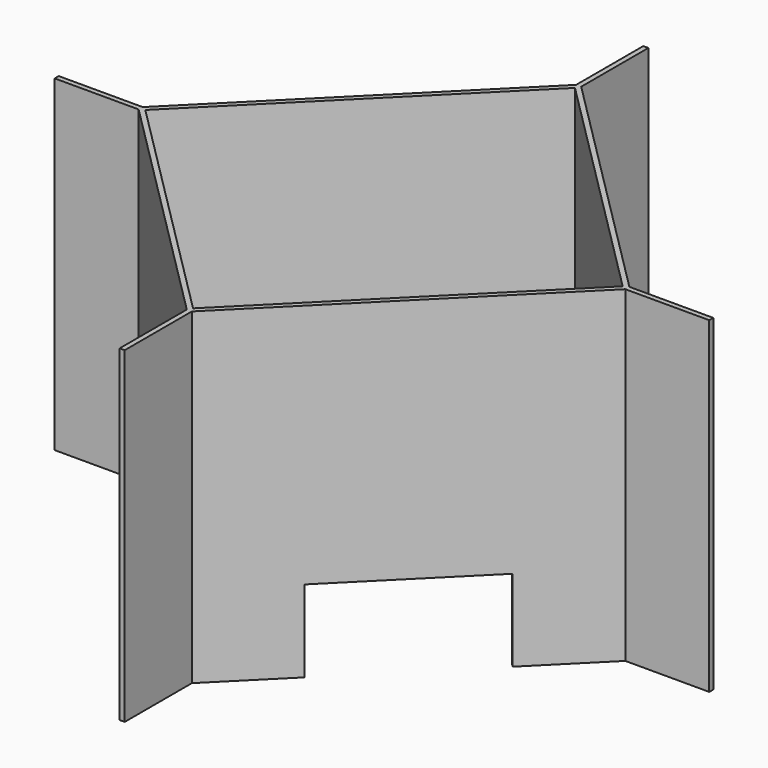
from build123d import *

# Parameters (mm, degrees)
F1_DEPTH        = 101.6
F2_T            = -1.5748
F4_DEPTH        = 101.6
F4_COPIES_COUNT = 4
F6_W            = 50.8
F6_H            = 25.4
F7_DEPTH        = 1.5748
F7_COPIES_COUNT = 4


# Not quite as in the source:
# - a pattern or mirror of a feature is missing from the dataset's text; its kind, count and spacing are read off the source's solid


with BuildPart() as f1:
    # F0 (on Top) → F1 (new body)
    with BuildSketch(Plane.XY):
        Polygon((76.3321770291, 0), (0, 76.3321770291), (-76.3321770291, 0), (0, -76.3321770291), align=None)
    extrude(amount=F1_DEPTH)

    # F2
    f2_openings = [f1.faces().sort_by_distance(p)[0] for p in [
        (0, 0, 101.6),
        (0, 0, 0),
    ]]
    offset(amount=F2_T, openings=f2_openings)

    # F3 (on face) → F4 (join, through all)
    with BuildSketch(Plane.XY.offset(101.6)):
        Polygon((-101.6, -0.7874), (-75.5447770291, -0.7874), (-76.3321770291, 0), (-75.5447770291, 0.7874), (-101.6, 0.7874), align=None)
        Polygon((-75.5447770291, -0.7874), (-73.3176735111, -0.7874), (-74.1050735111, 0), (-73.3176735111, 0.7874), (-75.5447770291, 0.7874), (-76.3321770291, 0), align=None)
    f4 = extrude(amount=-F4_DEPTH)

    # F4_copies: F4 ×4 about axis
    f4_copies_axis = Axis((0, 0, 0), (0, 0, 1))
    for i in range(1, F4_COPIES_COUNT):
        add(f4.rotate(f4_copies_axis, i * 360 / F4_COPIES_COUNT))

    # F6 (on face) → F7 (cut, through all)
    with BuildSketch(Plane(origin=(38.1660885145, -38.1660885145, 0), x_dir=(0.7071067812, 0.7071067812, 0), z_dir=(0.7071067812, -0.7071067812, 0))):
        with Locations((0, 12.7)):
            Rectangle(F6_W, F6_H)
    f7 = extrude(amount=-F7_DEPTH, mode=Mode.SUBTRACT)

    # F7_copies: F7 ×4 about axis
    f7_copies_axis = Axis((0, 0, 0), (0, 0, 1))
    for i in range(1, F7_COPIES_COUNT):
        add(f7.rotate(f7_copies_axis, i * 360 / F7_COPIES_COUNT), mode=Mode.SUBTRACT)


solid = f1.part
